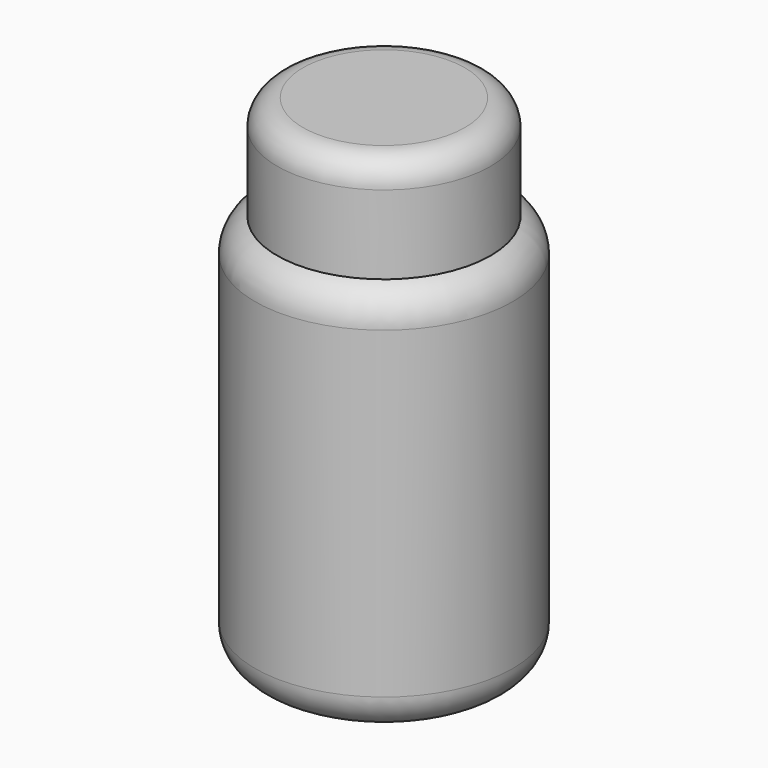
from build123d import *

# Parameters (mm, degrees)
F0_R     = 25.065
F1_DEPTH = 38.13
F2_R     = 20.75
F3_DEPTH = 20.3
F5_R     = 5


# Not quite as in the source:
# - a fillet or chamfer that OpenCascade refuses, or shapes differently, is made with other operations: its cross-section is extruded or revolved along the edge and cut away or added


with BuildPart() as f1:
    # F0 (on Top) → F1 (new body, symmetric)
    with BuildSketch(Plane.XY):
        Circle(F0_R)
    extrude(amount=F1_DEPTH, both=True)

    # F2 (on face) → F3 (join)
    with BuildSketch(Plane.XY.offset(38.13)):
        Circle(F2_R)
    extrude(amount=F3_DEPTH)

    # F4: fillet of radius 7 on 2 edges, made by hand

    # F4_s1 → F4_t2 (revolve, cut)
    with BuildSketch(Plane.XZ):
        with BuildLine():
            ThreePointArc((25.065, 31.6654215141), (23.8871559581, 35.5516150245), (20.75, 38.13))
            Line((20.75, 38.13), (25.065, 38.13))
            Line((25.065, 38.13), (25.065, 31.6654215141))
        make_face()
    revolve(axis=Axis((0, 0, 38.13), (0, 0, 1)), mode=Mode.SUBTRACT)

    # F4_s3 → F4_t4 (revolve, cut)
    with BuildSketch(Plane.XZ):
        with BuildLine():
            ThreePointArc((25.065, -31.13), (23.0147474683, -36.0797474683), (18.065, -38.13))
            Line((18.065, -38.13), (25.065, -38.13))
            Line((25.065, -38.13), (25.065, -31.13))
        make_face()
    revolve(axis=Axis((0, 0, -38.13), (0, 0, 1)), mode=Mode.SUBTRACT)

    # F5
    f5_edges = [f1.edges().sort_by_distance(p)[0] for p in [
        (-20.75, 0, 58.43),
    ]]
    fillet(f5_edges, radius=F5_R)


solid = f1.part
